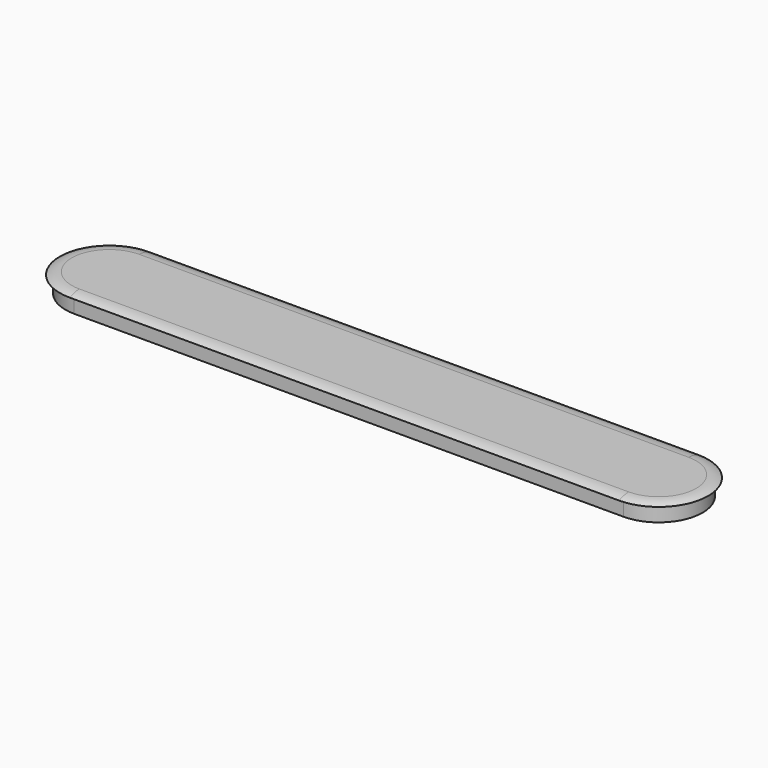
from build123d import *

# Parameters (mm, degrees)
F1_DEPTH    = 3
F3_DEPTH    = 0.5
F4_T1_DEPTH = 100
F4_T4_ANGLE = 180
F4_T6_ANGLE = 180


# Not quite as in the source:
# - a fillet or chamfer that OpenCascade refuses, or shapes differently, is made with other operations: its cross-section is extruded or revolved along the edge and cut away or added


with BuildPart() as f1:
    # F0 (on Top) → F1 (new body)
    with BuildSketch(Plane.XY):
        with BuildLine():
            Line((71.8090593611, 7.9999995343), (-28.1909406389, 7.9999995343))
            ThreePointArc((-28.1909406389, 7.9999995343), (-36.1909406389, -4.657e-07), (-28.1909406389, -8.0000004657))
            Line((-28.1909406389, -8.0000004657), (71.8090593611, -8.0000004657))
            ThreePointArc((71.8090593611, -8.0000004657), (79.8090593611, -4.657e-07), (71.8090593611, 7.9999995343))
        make_face()
    extrude(amount=F1_DEPTH)

    # F2 (on face) → F3 (join)
    with BuildSketch(Plane.XY.offset(3)):
        with BuildLine():
            Line((71.8090593611, 8.9999995343), (-28.1909406389, 8.9999995343))
            ThreePointArc((-28.1909406389, 8.9999995343), (-37.1909406389, -4.657e-07), (-28.1909406389, -9.0000004657))
            Line((-28.1909406389, -9.0000004657), (71.8090593611, -9.0000004657))
            ThreePointArc((71.8090593611, -9.0000004657), (80.8090593611, -4.657e-07), (71.8090593611, 8.9999995343))
        make_face()
        with BuildLine():
            Line((-28.1909406389, 7.9999995343), (71.8090593611, 7.9999995343))
            ThreePointArc((71.8090593611, 7.9999995343), (79.8090593611, -4.657e-07), (71.8090593611, -8.0000004657))
            Line((71.8090593611, -8.0000004657), (-28.1909406389, -8.0000004657))
            ThreePointArc((-28.1909406389, -8.0000004657), (-36.1909406389, -4.657e-07), (-28.1909406389, 7.9999995343))
        make_face(mode=Mode.SUBTRACT)
        with BuildLine():
            ThreePointArc((71.8090593611, -8.0000004657), (79.8090593611, -4.657e-07), (71.8090593611, 7.9999995343))
            Line((71.8090593611, 7.9999995343), (-28.1909406389, 7.9999995343))
            ThreePointArc((-28.1909406389, 7.9999995343), (-36.1909406389, -4.657e-07), (-28.1909406389, -8.0000004657))
            Line((-28.1909406389, -8.0000004657), (71.8090593611, -8.0000004657))
        make_face()
    extrude(amount=F3_DEPTH)

    # F4: fillet of radius 5 on 4 edges, made by hand

    # F4_s2 → F4_t1 (cut)
    with BuildSketch(Plane.YZ.offset(-28.1909406389)):
        with BuildLine():
            ThreePointArc((-9.0000004657, 3), (-7.9385849826, 3.3733971724), (-6.8205509939, 3.5))
            Line((-6.8205509939, 3.5), (-9.0000004657, 3.5))
            Line((-9.0000004657, 3.5), (-9.0000004657, 3))
        make_face()
        with BuildLine():
            ThreePointArc((8.9999995343, 3), (7.9385840513, 3.3733971724), (6.8205500626, 3.5))
            Line((6.8205500626, 3.5), (8.9999995343, 3.5))
            Line((8.9999995343, 3.5), (8.9999995343, 3))
        make_face()
    extrude(amount=F4_T1_DEPTH, mode=Mode.SUBTRACT)

    # F4_s3 → F4_t4 (revolve, cut)
    with BuildSketch(Plane.YZ.offset(-28.1909406389)):
        with BuildLine():
            ThreePointArc((8.9999995343, 3), (7.9385840513, 3.3733971724), (6.8205500626, 3.5))
            Line((6.8205500626, 3.5), (8.9999995343, 3.5))
            Line((8.9999995343, 3.5), (8.9999995343, 3))
        make_face()
    revolve(axis=Axis((-28.1909406389, -4.657e-07, 3.5), (0, 0, 1)), revolution_arc=F4_T4_ANGLE, mode=Mode.SUBTRACT)

    # F4_s5 → F4_t6 (revolve, cut)
    with BuildSketch(Plane.YZ.offset(71.8090593611)):
        with BuildLine():
            ThreePointArc((-6.8205509939, 3.5), (-7.9385849826, 3.3733971724), (-9.0000004657, 3))
            Line((-9.0000004657, 3), (-9.0000004657, 3.5))
            Line((-9.0000004657, 3.5), (-6.8205509939, 3.5))
        make_face()
    revolve(axis=Axis((71.8090593611, -4.657e-07, 3.5), (0, 0, 1)), revolution_arc=F4_T6_ANGLE, mode=Mode.SUBTRACT)


solid = f1.part
